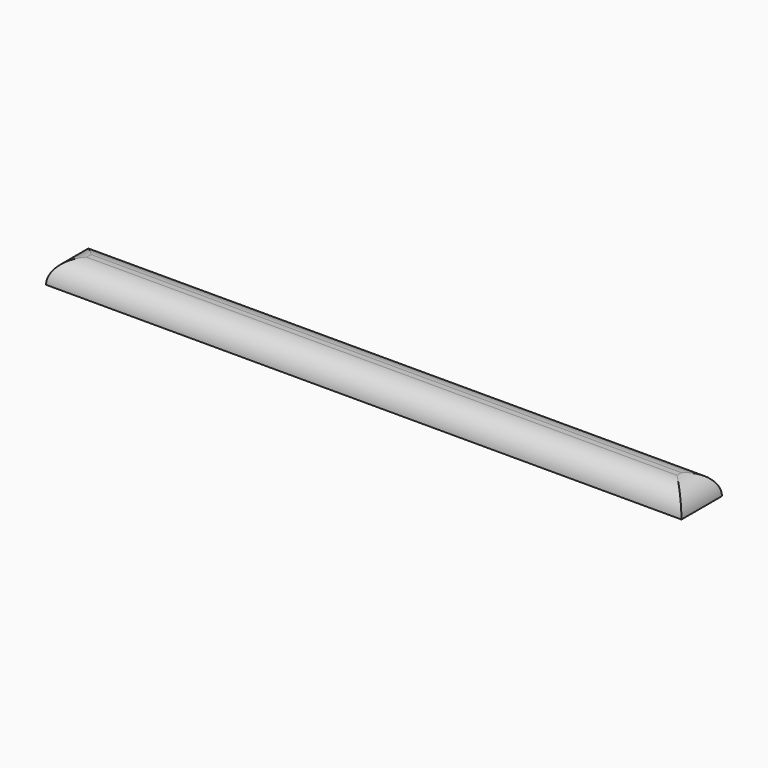
from build123d import *

# Parameters (mm, degrees)
F0_W     = 113.008
F0_H     = 9
F1_DEPTH = 4
F2_R     = 3.99999


# Not quite as in the source:
# - a fillet or chamfer is up to 0.001 mm smaller than in the source, because OpenCascade refuses the exact size


with BuildPart() as f1:
    # F0 (on Top) → F1 (new body)
    with BuildSketch(Plane.XY):
        Rectangle(F0_W, F0_H)
    extrude(amount=F1_DEPTH)

    # F2 (radius 4 in the source; OpenCascade refuses exactly that, so slightly less here)
    f2_edges = [f1.edges().sort_by_distance(p)[0] for p in [
        (0, 4.5, 4),
        (0, -4.5, 4),
        (-56.504, 0, 4),
        (56.504, 0, 4),
    ]]
    fillet(f2_edges, radius=F2_R)


solid = f1.part
